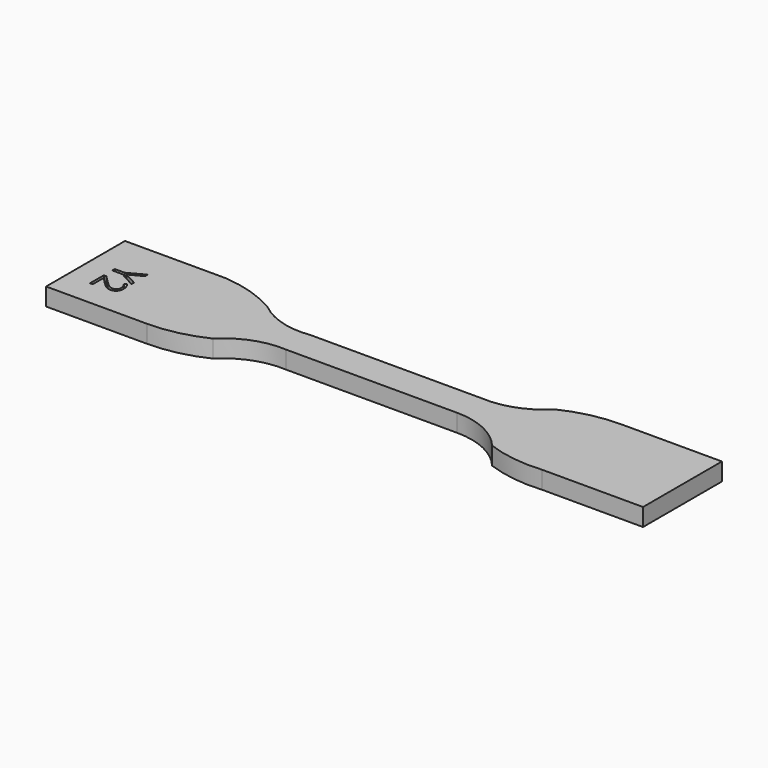
from build123d import *

# Parameters (mm, degrees)
F1_DEPTH     = 3.4
F2_TEXT_SIZE = 7.0564552314
F3_DEPTH     = 1


# Not quite as in the source:
# - Text() gives the source's letters only with a copy of the font that has no kerning and outlines rounded to 1/6400 em; it was checked with that copy


with BuildPart() as f1:
    # F0 (on Top) → F1 (new body)
    with BuildSketch(Plane.XY):
        with BuildLine():
            Line((-14.4320548165, 19.7811394548), (-33.8720548165, 19.7811394548))
            Line((-33.8720548165, 19.7811394548), (-33.8720548165, 0.7811394548))
            Line((-33.8720548165, 0.7811394548), (-14.4320548165, 0.7811394548))
            ThreePointArc((-14.4320548165, 0.7811394548), (-8.9053122052, 1.3996892086), (-3.6520548165, 3.2247301661))
            ThreePointArc((-3.6520548165, 3.2247301661), (1.3014698263, 6.4128780055), (7.1279451835, 7.2811394548))
            Line((7.1279451835, 7.2811394548), (40.1279451835, 7.2811394548))
            ThreePointArc((40.1279451835, 7.2811394548), (46.0837574042, 5.9511158081), (50.9079451835, 2.2137538538))
            ThreePointArc((50.9079451835, 2.2137538538), (56.2191047011, 0.9041953221), (61.6879451835, 0.7811394548))
            Line((61.6879451835, 0.7811394548), (81.1279451835, 0.7811394548))
            Line((81.1279451835, 0.7811394548), (81.1279451835, 19.7811394548))
            Line((81.1279451835, 19.7811394548), (61.6879451835, 19.7811394548))
            ThreePointArc((61.6879451835, 19.7811394548), (56.1612025723, 19.162589701), (50.9079451835, 17.3375487435))
            ThreePointArc((50.9079451835, 17.3375487435), (45.9544205407, 14.1494009041), (40.1279451835, 13.2811394548))
            Line((40.1279451835, 13.2811394548), (7.1279451835, 13.2811394548))
            ThreePointArc((7.1279451835, 13.2811394548), (1.4167452884, 13.6925537245), (-3.6520548165, 16.3560723447))
            ThreePointArc((-3.6520548165, 16.3560723447), (-8.8458057958, 18.686276846), (-14.4320548165, 19.7811394548))
        make_face()
    extrude(amount=F1_DEPTH)

    # F2 (on face) → F3 (cut)
    with BuildSketch(Plane.XY.offset(3.4)):
        with Locations(Location((-29.3720550835, 13.353464842), (0, 0, -90))):
            Text('Y2', F2_TEXT_SIZE, font='Open Sans', text_align=(TextAlign.LEFT, TextAlign.BOTTOM))
    extrude(amount=-F3_DEPTH, mode=Mode.SUBTRACT)


solid = f1.part
